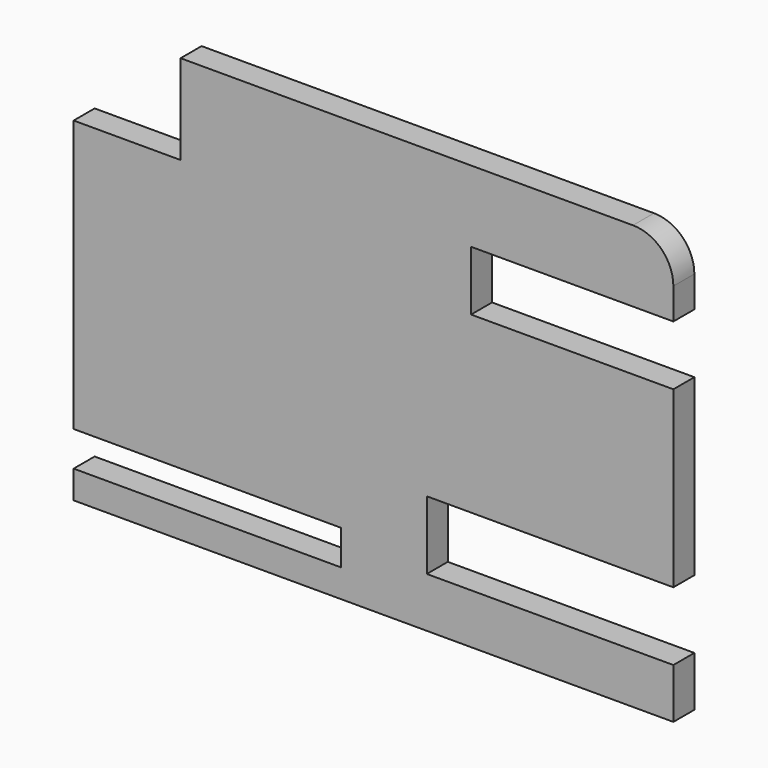
from build123d import *

# Parameters (mm, degrees)
F1_DEPTH = 13
F2_W     = 132.4155251533
F2_H     = 17.2680690885
F3_DEPTH = 13
F4_W     = 100.1826098412
F4_H     = 29.5549705625
F5_DEPTH = 13
F6_W     = 122.0997741669
F6_H     = 33.8719934225
F7_DEPTH = 13


# Not quite as in the source:
# - the program builds the solid bodies; features that only make, move or delete a surface that nothing else refers to are left out


with BuildPart() as f1:
    # F0 (on Front) → F1 (new body)
    with BuildSketch(Plane.XZ):
        with BuildLine():
            Line((144.5844748467, 101.5557457248), (-79.4445127249, 101.5557457248))
            Line((-79.4445127249, 101.5557457248), (-79.4445127249, 57.1600347757))
            Line((-79.4445127249, 57.1600347757), (-132.4155251533, 57.1600347757))
            Line((-132.4155251533, 57.1600347757), (-132.4155251533, -108.4442542752))
            Line((-132.4155251533, -108.4442542752), (164.5844748467, -108.4442542752))
            Line((164.5844748467, -108.4442542752), (164.5844748467, 81.5557457248))
            ThreePointArc((164.5844748467, 81.5557457248), (158.7266104705, 95.6978813486), (144.5844748467, 101.5557457248))
        make_face()
    extrude(amount=F1_DEPTH)

    # F2 (on face) → F3 (cut)
    with BuildSketch(Plane.XZ.offset(13)):
        with Locations((-66.2077625766, -85.9657116234)):
            Rectangle(F2_W, F2_H)
    extrude(amount=-F3_DEPTH, mode=Mode.SUBTRACT)

    # F4 (on face) → F5 (cut)
    with BuildSketch(Plane.XZ.offset(13)):
        with Locations((114.4931699261, 51.3486675918)):
            Rectangle(F4_W, F4_H)
    extrude(amount=-F5_DEPTH, mode=Mode.SUBTRACT)

    # F6 (on face) → F7 (cut)
    with BuildSketch(Plane.XZ.offset(13)):
        with Locations((103.5345877632, -66.7051747441)):
            Rectangle(F6_W, F6_H)
    extrude(amount=-F7_DEPTH, mode=Mode.SUBTRACT)


solid = f1.part
